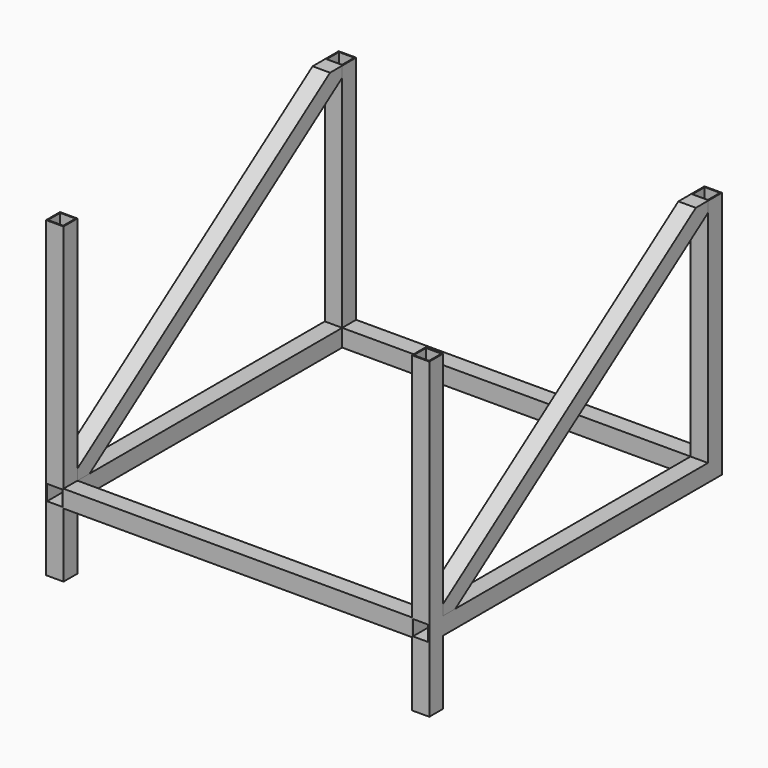
from build123d import *

# Parameters (mm, degrees)
F0_W      = 25.4
F0_H      = 25.4
F0_W_2    = 22.352
F0_H_2    = 22.352
F1_DEPTH  = 533.4
F3_W      = 25.4
F3_H      = 25.4
F3_W_2    = 22.352
F3_H_2    = 22.352
F4_DEPTH  = 508
F6_W      = 25.4
F6_H      = 25.4
F6_W_2    = 22.352
F6_H_2    = 22.352
F7_DEPTH  = 336.55
F8_W      = 25.4
F8_H      = 25.4
F8_W_2    = 22.352
F8_H_2    = 22.352
F9_DEPTH  = 336.55
F10_W     = 25.4
F10_H     = 25.4
F10_W_2   = 22.352
F10_H_2   = 22.352
F11_DEPTH = 336.55
F12_W     = 25.4
F12_H     = 25.4
F12_W_2   = 22.352
F12_H_2   = 22.352
F13_DEPTH = 336.55
F14_W     = 25.4
F14_H     = 25.4
F14_W_2   = 22.352
F14_H_2   = 22.352
F15_DEPTH = 93.98
F16_W     = 25.4
F16_H     = 25.4
F16_W_2   = 22.352
F16_H_2   = 22.352
F17_DEPTH = 93.98
F19_DEPTH = 25.4


with BuildPart() as f1:
    # F0 (on Front) → F1 (new body)
    with BuildSketch(Plane.XZ):
        with Locations((33.4044629708, 39.9714800462)):
            Rectangle(F0_W, F0_H)
        with Locations((33.4044629708, 39.9714800462)):
            Rectangle(F0_W_2, F0_H_2, mode=Mode.SUBTRACT)
    extrude(amount=F1_DEPTH)


with BuildPart() as f2_1:
    # F2: copy of F1
    add(f1.part.moved(Location((533.4, 0, 0))))

    # F8 (on face) → F9 (join)
    with BuildSketch(Plane.XY.offset(52.6714800462)):
        with Locations((566.8044629708, -520.7)):
            Rectangle(F8_W, F8_H)
        with Locations((566.8044629708, -520.7)):
            Rectangle(F8_W_2, F8_H_2, mode=Mode.SUBTRACT)
    extrude(amount=F9_DEPTH)

    # F10 (on face) → F11 (join)
    with BuildSketch(Plane.XY.offset(52.6714800462)):
        with Locations((566.8044629708, -12.7)):
            Rectangle(F10_W, F10_H)
        with Locations((566.8044629708, -12.7)):
            Rectangle(F10_W_2, F10_H_2, mode=Mode.SUBTRACT)
    extrude(amount=F11_DEPTH)

    # F16 (on face) → F17 (join)
    with BuildSketch(Plane(origin=(0, 0, 27.2714800462), x_dir=(1, 0, 0), z_dir=(0, 0, -1))):
        with Locations((566.8044629708, 520.7)):
            Rectangle(F16_W, F16_H)
        with Locations((566.8044629708, 520.7)):
            Rectangle(F16_W_2, F16_H_2, mode=Mode.SUBTRACT)
    extrude(amount=F17_DEPTH)


with BuildPart() as f4:
    # F3 (on face) → F4 (new body)
    with BuildSketch(Plane(origin=(554.1044629708, 0, 0), x_dir=(0, -1, 0), z_dir=(-1, 0, 0))):
        with Locations((520.7, 39.9714800462)):
            Rectangle(F3_W, F3_H)
        with Locations((520.7, 39.9714800462)):
            Rectangle(F3_W_2, F3_H_2, mode=Mode.SUBTRACT)
    extrude(amount=F4_DEPTH)


with BuildPart() as f5_1:
    # F5: copy of F4
    add(f4.part.moved(Location((0, 508, 0))))


with BuildPart() as f1_1:
    add(f1.part)

    # F6 (on face) → F7 (join)
    with BuildSketch(Plane.XY.offset(52.6714800462)):
        with Locations((33.4044629708, -520.7)):
            Rectangle(F6_W, F6_H)
        with Locations((33.4044629708, -520.7)):
            Rectangle(F6_W_2, F6_H_2, mode=Mode.SUBTRACT)
    extrude(amount=F7_DEPTH)

    # F12 (on face) → F13 (join)
    with BuildSketch(Plane.XY.offset(52.6714800462)):
        with Locations((33.4044629708, -12.7)):
            Rectangle(F12_W, F12_H)
        with Locations((33.4044629708, -12.7)):
            Rectangle(F12_W_2, F12_H_2, mode=Mode.SUBTRACT)
    extrude(amount=F13_DEPTH)

    # F14 (on face) → F15 (join)
    with BuildSketch(Plane(origin=(0, 0, 27.2714800462), x_dir=(1, 0, 0), z_dir=(0, 0, -1))):
        with Locations((33.4044629708, 520.7)):
            Rectangle(F14_W, F14_H)
        with Locations((33.4044629708, 520.7)):
            Rectangle(F14_W_2, F14_H_2, mode=Mode.SUBTRACT)
    extrude(amount=F15_DEPTH)


with BuildPart() as f19:
    # F18 (on face) → F19 (new body)
    with BuildSketch(Plane(origin=(20.7044629708, 0, 0), x_dir=(0, -1, 0), z_dir=(-1, 0, 0))):
        Polygon((25.4, 389.2214800462), (25.4, 373.7382959211), (485.7976982357, 52.6714800462), (508, 52.6714800462), (508, 68.1546641712), (47.6023017643, 389.2214800462), align=None)
    extrude(amount=-F19_DEPTH)


with BuildPart() as f20_1:
    # F20: copy of F19
    add(f19.part.moved(Location((533.4, 0, 0))))


solid = Compound([f2_1.part, f4.part, f5_1.part, f1_1.part, f19.part, f20_1.part])
